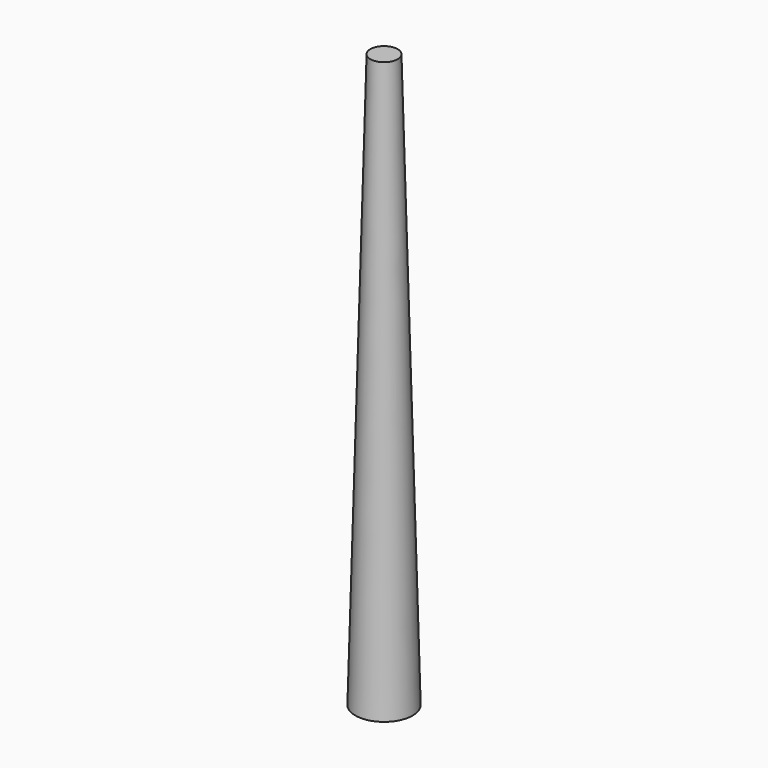
from build123d import *

# Parameters (mm, degrees)
F0_R     = 19.05
F1_DEPTH = 381
F1_TAPER = 1.5


with BuildPart() as f1:
    # F0 (on Top) → F1 (new body)
    with BuildSketch(Plane.XY):
        Circle(F0_R)
    extrude(amount=F1_DEPTH, taper=F1_TAPER)


solid = f1.part
